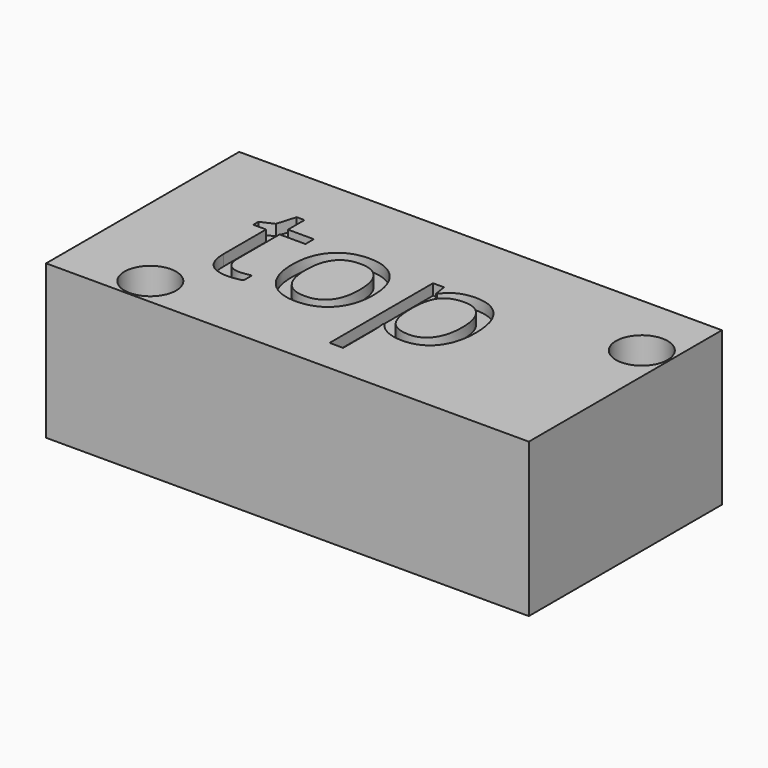
from build123d import *

# Parameters (mm, degrees)
F0_W         = 44
F0_H         = 22
F1_DEPTH     = 14
F2_R         = 1.25
F3_DEPTH     = 14
F4_TEXT_SIZE = 15.1962190608
F5_DEPTH     = 1
F6_R         = 2.35
F7_DEPTH     = 12


# Not quite as in the source:
# - Text() gives the source's letters only with a copy of the font that has no kerning and outlines rounded to 1/6400 em; it was checked with that copy


with BuildPart() as f1:
    # F0 (on Top) → F1 (new body)
    with BuildSketch(Plane.XY):
        Rectangle(F0_W, F0_H)
    extrude(amount=F1_DEPTH)

    # F2 (on face) → F3 (cut, through all)
    with BuildSketch(Plane.XY.offset(14)):
        with Locations((19.5, 5)):
            Circle(F2_R)
        with Locations((-14.5, -8.5)):
            Circle(F2_R)
    extrude(amount=-F3_DEPTH, mode=Mode.SUBTRACT)

    # F4 (on face) → F5 (cut)
    with BuildSketch(Plane.XY.offset(14)):
        with Locations((-14.4310286269, -4.3200906366)):
            Text('top', F4_TEXT_SIZE, font='Open Sans', text_align=(TextAlign.LEFT, TextAlign.BOTTOM))
    extrude(amount=-F5_DEPTH, mode=Mode.SUBTRACT)

    # F6 (on face) → F7 (cut)
    with BuildSketch(Plane.XY.offset(14)):
        with Locations((-14.5, -8.5)):
            Circle(F6_R)
        with Locations((19.5, 5)):
            Circle(F6_R)
    extrude(amount=-F7_DEPTH, mode=Mode.SUBTRACT)


solid = f1.part
